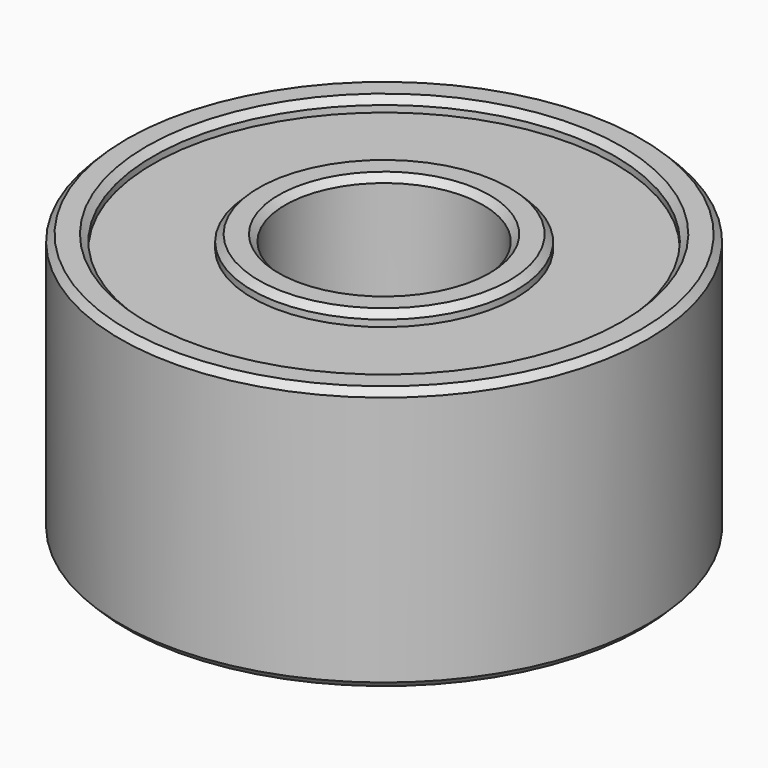
from build123d import *

# Parameters (mm, degrees)
F0_R      = 2
F0_R_2    = 1.5
F1_DEPTH  = 4
F0_R_3    = 4
F0_R_4    = 3.5
F2_START  = 0.2
F2_DEPTH  = 3.6
F3_SIZE   = 0.1
F3_2_SIZE = 0.1


with BuildPart() as f1:
    # F0 (on Top) → F1 (new body)
    with BuildSketch(Plane.XY):
        Circle(F0_R)
        Circle(F0_R_2, mode=Mode.SUBTRACT)
    extrude(amount=F1_DEPTH)

    # F3
    f3_edges = [f1.edges().sort_by_distance(p)[0] for p in [
        (-2, 0, 0),
        (-1.5, 0, 0),
        (-2, 0, 4),
        (-1.5, 0, 4),
    ]]
    chamfer(f3_edges, length=F3_SIZE)


with BuildPart() as f1b:
    # F0 (on Top) → F1, piece 2 (new body)
    with BuildSketch(Plane.XY):
        Circle(F0_R_3)
        Circle(F0_R_4, mode=Mode.SUBTRACT)
    extrude(amount=F1_DEPTH)

    # F3#2
    f3_2_edges = [f1b.edges().sort_by_distance(p)[0] for p in [
        (-4, 0, 4),
        (-3.5, 0, 4),
        (-4, 0, 0),
        (-3.5, 0, 0),
    ]]
    chamfer(f3_2_edges, length=F3_2_SIZE)


with BuildPart() as f2:
    # F0 (on Top) → F2 (new body)
    with BuildSketch(Plane.XY.offset(F2_START)):
        Circle(F0_R_4)
        Circle(F0_R, mode=Mode.SUBTRACT)
    extrude(amount=F2_DEPTH)


solid = Compound([f1.part, f1b.part, f2.part])
